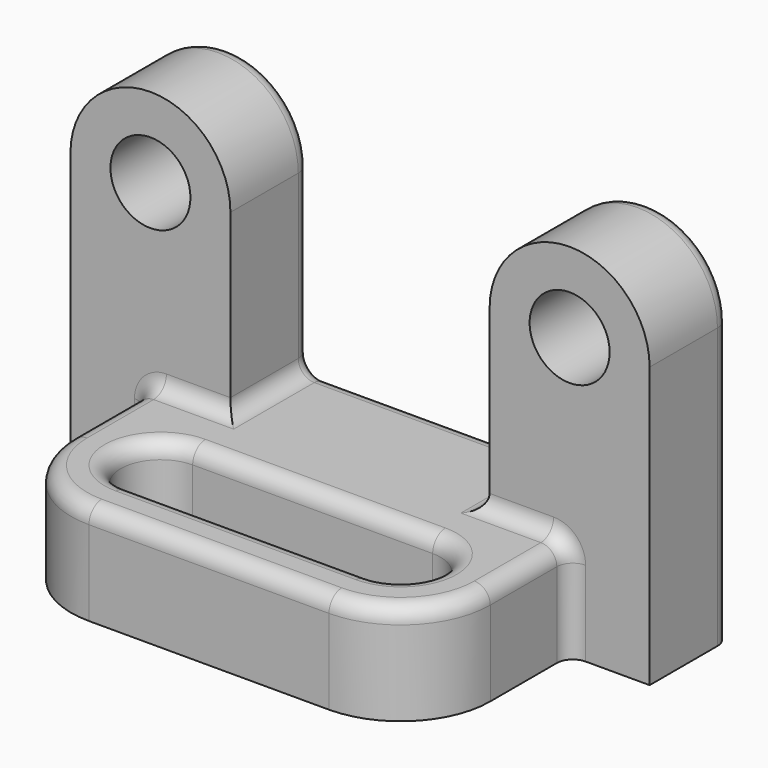
from build123d import *

# Parameters (mm, degrees)
F1_DEPTH = 16.002
F3_DEPTH = 16.002
F4_R     = 2.54


with BuildPart() as f1:
    # F0 (on Top) → F1 (new body)
    with BuildSketch(Plane.XY):
        with BuildLine():
            ThreePointArc((38.1, -7.874), (48.1578868556, -3.7078868556), (52.324, 6.35))
            Line((52.324, 6.35), (52.324, 38.1))
            Line((52.324, 38.1), (-14.224, 38.1))
            Line((-14.224, 38.1), (-14.224, 6.35))
            ThreePointArc((-14.224, 6.35), (-10.0578868556, -3.7078868556), (0, -7.874))
            Line((0, -7.874), (38.1, -7.874))
        make_face()
        with BuildLine():
            Line((38.1, 0), (0, 0))
            ThreePointArc((0, 0), (-6.35, 6.35), (0, 12.7))
            Line((0, 12.7), (38.1, 12.7))
            ThreePointArc((38.1, 12.7), (44.45, 6.35), (38.1, 0))
        make_face(mode=Mode.SUBTRACT)
    extrude(amount=F1_DEPTH)

    # F2 (on face) → F3 (join)
    with BuildSketch(Plane(origin=(0, 38.1, 0), x_dir=(-1, 0, 0), z_dir=(0, 1, 0))):
        with BuildLine():
            Line((26.924, 0), (26.924, 44.45))
            Line((26.924, 44.45), (20.574, 44.45))
            ThreePointArc((20.574, 44.45), (14.224, 38.1), (7.874, 44.45))
            Line((7.874, 44.45), (1.524, 44.45))
            Line((1.524, 44.45), (1.524, 0))
            Line((1.524, 0), (26.924, 0))
        make_face()
        with BuildLine():
            Line((20.574, 44.45), (26.924, 44.45))
            ThreePointArc((26.924, 44.45), (14.224, 57.15), (1.524, 44.45))
            Line((1.524, 44.45), (7.874, 44.45))
            ThreePointArc((7.874, 44.45), (14.224, 50.8), (20.574, 44.45))
        make_face()
        with BuildLine():
            Line((-39.624, 0), (-39.624, 44.45))
            Line((-39.624, 44.45), (-45.974, 44.45))
            ThreePointArc((-45.974, 44.45), (-52.324, 38.1), (-58.674, 44.45))
            Line((-58.674, 44.45), (-65.024, 44.45))
            Line((-65.024, 44.45), (-65.024, 0))
            Line((-65.024, 0), (-39.624, 0))
        make_face()
        with BuildLine():
            Line((-45.974, 44.45), (-39.624, 44.45))
            ThreePointArc((-39.624, 44.45), (-52.324, 57.15), (-65.024, 44.45))
            Line((-65.024, 44.45), (-58.674, 44.45))
            ThreePointArc((-58.674, 44.45), (-52.324, 50.8), (-45.974, 44.45))
        make_face()
    extrude(amount=-F3_DEPTH)

    # F4
    f4_edges = [f1.edges().sort_by_distance(p)[0] for p in [
        (52.324, 14.224, 16.002),
        (-10.057887, -3.707887, 16.002),
        (-14.224, 14.224, 16.002),
        (-7.874, 22.098, 16.002),
        (-1.524, 30.099, 16.002),
        (19.05, 38.1, 16.002),
        (39.624, 30.099, 16.002),
        (45.974, 22.098, 16.002),
        (48.157887, -3.707887, 16.002),
        (19.05, -7.874, 16.002),
        (44.45, 6.35, 16.002),
        (19.05, 12.7, 16.002),
        (19.05, 0, 16.002),
        (-6.35, 6.35, 16.002),
        (52.324, 22.098, 8.001),
        (52.324, 38.1, 57.15),
        (65.024, 38.1, 22.225),
        (39.624, 38.1, 30.226),
        (-1.524, 38.1, 30.226),
        (-14.224, 38.1, 57.15),
        (-26.924, 38.1, 22.225),
        (-14.224, 22.098, 8.001),
    ]]
    fillet(f4_edges, radius=F4_R)


solid = f1.part
